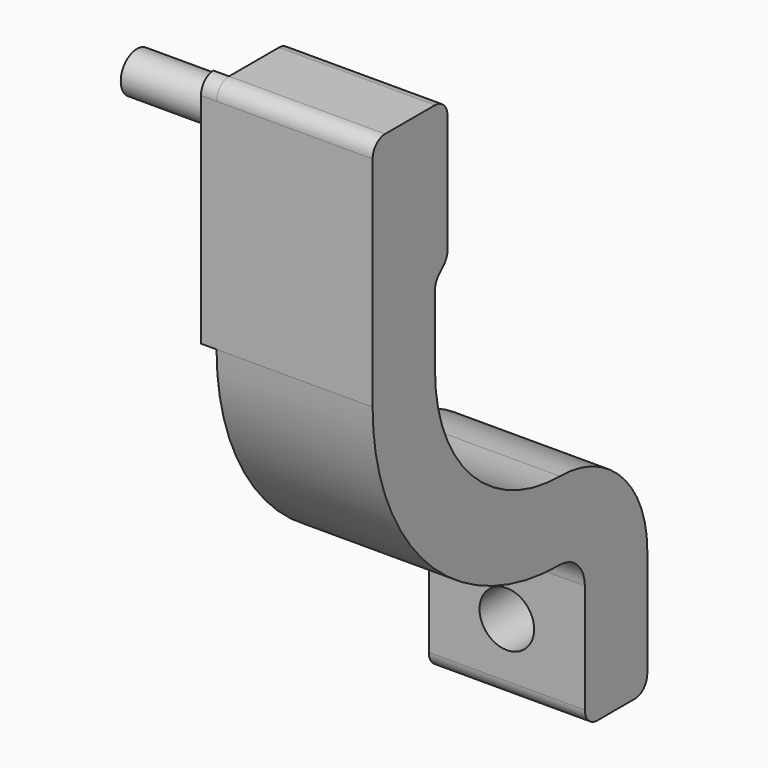
from build123d import *

# Parameters (mm, degrees)
F2_DEPTH  = 12.7
F3_R      = 12.7
F4_R      = 19.05
F5_R      = 8.88999
F6_R      = 2.53999
F7_R      = 1.27
F8_R      = 2.2225
F9_DEPTH  = 6.35
F10_R     = 1.651
F11_DEPTH = 9.525
F13_DEPTH = 1.27


# Not quite as in the source:
# - a fillet or chamfer is up to 0.001 mm smaller than in the source, because OpenCascade refuses the exact size


with BuildPart() as f2:
    # F1 (on Right) → F2 (new body)
    with BuildSketch(Plane.YZ):
        Polygon((-26.67, -19.05), (-26.67, 0), (-25.4, 1.27), (-25.4, 12.7), (-33.02, 12.7), (-33.02, -25.4), (-11.43, -25.4), (-11.43, -38.1), (-5.08, -38.1), (-5.08, -19.05), align=None)
    extrude(amount=F2_DEPTH)

    # F3
    f3_edges = [f2.edges().sort_by_distance(p)[0] for p in [
        (6.35, -26.67, -19.05),
    ]]
    fillet(f3_edges, radius=F3_R)

    # F4
    f4_edges = [f2.edges().sort_by_distance(p)[0] for p in [
        (6.35, -33.02, -25.4),
    ]]
    fillet(f4_edges, radius=F4_R)

    # F5 (radius 8.89 in the source; OpenCascade refuses exactly that, so slightly less here)
    f5_edges = [f2.edges().sort_by_distance(p)[0] for p in [
        (6.35, -5.08, -19.05),
    ]]
    fillet(f5_edges, radius=F5_R)

    # F6 (radius 2.54 in the source; OpenCascade refuses exactly that, so slightly less here)
    f6_edges = [f2.edges().sort_by_distance(p)[0] for p in [
        (6.35, -11.43, -25.4),
    ]]
    fillet(f6_edges, radius=F6_R)

    # F7
    f7_edges = [f2.edges().sort_by_distance(p)[0] for p in [
        (6.35, -26.67, 0),
        (6.35, -25.4, 1.27),
        (6.35, -25.4, 12.7),
        (6.35, -33.02, 12.7),
        (6.35, -11.43, -38.1),
        (6.35, -5.08, -38.1),
    ]]
    fillet(f7_edges, radius=F7_R)

    # F8 (on face) → F9 (cut)
    with BuildSketch(Plane.XZ.offset(11.43)):
        with Locations((6.35, -32.385)):
            Circle(F8_R)
    extrude(amount=-F9_DEPTH, mode=Mode.SUBTRACT)

    # F10 (on face) → F11 (join)
    with BuildSketch(Plane(origin=(0, 0, 0), x_dir=(0, -1, 0), z_dir=(-1, 0, 0))):
        with Locations((29.21, 8.89)):
            Circle(F10_R)
    extrude(amount=F11_DEPTH)

    # F12 (on face) → F13 (join)
    with BuildSketch(Plane(origin=(0, 0, 0), x_dir=(0, -1, 0), z_dir=(-1, 0, 0))):
        with BuildLine():
            Line((31.75, -6.35), (33.02, -6.35))
            Line((33.02, -6.35), (33.02, 11.43))
            ThreePointArc((33.02, 11.43), (32.6480256121, 12.3280256121), (31.75, 12.7))
            Line((31.75, 12.7), (31.75, -6.35))
        make_face()
    extrude(amount=F13_DEPTH)


solid = f2.part
